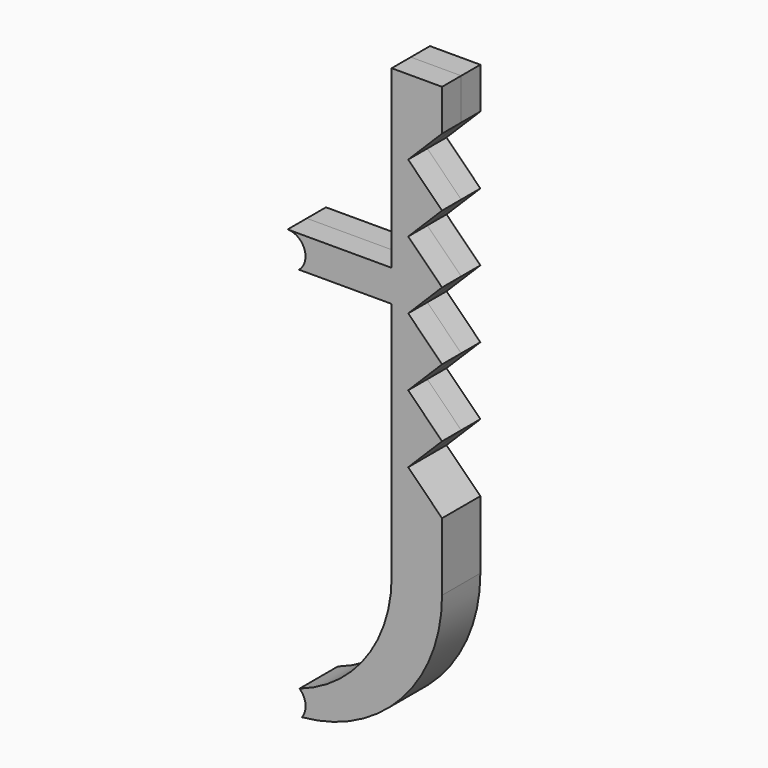
from build123d import *

# Parameters (mm, degrees)
F1_DEPTH = 3.175


# Not quite as in the source:
# - a feature names something its author has since deleted; it is built from what else it names


with BuildPart() as f1:
    # F0 (on Front) → F1 (new body, symmetric)
    with BuildSketch(Plane.XZ):
        Polygon((13.7837369962, 22.4047590313), (13.7837369962, -9.4272618645), (20.4636742089, -9.4272618645), (20.4636742089, -0.4338561879), (15.9735461484, 4.0562718726), (20.4636742089, 8.5463999331), (15.9735461484, 13.0365279937), (20.4636742089, 17.5266560542), (15.978414683, 22.0119155801), (20.4636742089, 26.497175106), (15.978414683, 30.9824346319), (20.4636742089, 35.4676941578), (15.9735461484, 39.9578222184), (20.4636742089, 44.4479502789), (20.4636742089, 49.9097465079), (13.7837369962, 49.9097465079), (13.7837369962, 26.6143454669), align=None)
        with BuildLine():
            ThreePointArc((1.5690815371, -26.4578800095), (2.166296426, -27.2647981392), (2.3779042983, -28.246126117))
            ThreePointArc((2.3779042983, -28.246126117), (2.2515693271, -29.011442898), (1.8859695789, -29.69555336))
            ThreePointArc((1.8859695789, -29.69555336), (15.116594907, -23.1743956519), (20.4636742089, -9.4272618645))
            Line((20.4636742089, -9.4272618645), (13.7837369962, -9.4272618645))
            ThreePointArc((13.7837369962, -9.4272618645), (10.4143723985, -19.9062857024), (1.5690815371, -26.4578800095))
        make_face()
        with BuildLine():
            Line((1.5079542983, 22.4047590313), (13.7837369962, 22.4047590313))
            Line((13.7837369962, 22.4047590313), (13.7837369962, 26.6143454669))
            Line((13.7837369962, 26.6143454669), (-0.0033457017, 26.6143454669))
            ThreePointArc((-0.0033457017, 26.6143454669), (1.6712163547, 25.9118815011), (2.363628681, 24.2331382585))
            ThreePointArc((2.363628681, 24.2331382585), (2.1391272177, 23.2237883133), (1.5079542983, 22.4047590313))
        make_face()
    extrude(amount=F1_DEPTH, both=True)


solid = f1.part
